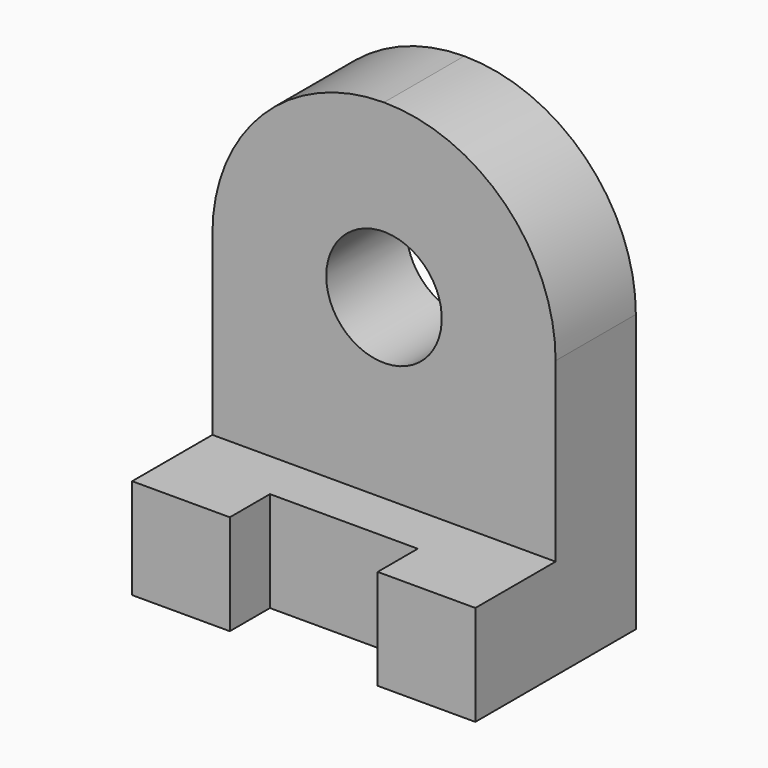
from build123d import *

# Parameters (mm, degrees)
F0_W     = 66.04
F0_H     = 86.36
F1_DEPTH = 19.304
F2_R     = 33.01999
F3_W     = 66.04
F3_H     = 19.304
F4_DEPTH = 19.304
F5_W     = 66.04
F5_H     = 19.304
F6_DEPTH = 9.652
F7_W     = 18.796
F7_H     = 19.304
F8_DEPTH = 9.652
F10_D    = 22.225


# Not quite as in the source:
# - a fillet or chamfer is up to 0.001 mm smaller than in the source, because OpenCascade refuses the exact size


with BuildPart() as f1:
    # F0 (on Front) → F1 (new body)
    with BuildSketch(Plane.XZ):
        with Locations((33.02, 43.18)):
            Rectangle(F0_W, F0_H)
    extrude(amount=F1_DEPTH)

    # F2 (radius 33.02 in the source; OpenCascade refuses exactly that, so slightly less here)
    f2_edges = [f1.edges().sort_by_distance(p)[0] for p in [
        (66.04, -9.652, 86.36),
        (0, -9.652, 86.36),
    ]]
    fillet(f2_edges, radius=F2_R)

    # F3 (on Front) → F4 (join)
    with BuildSketch(Plane.XZ):
        with Locations((33.02, 9.652)):
            Rectangle(F3_W, F3_H)
    extrude(amount=F4_DEPTH)

    # F5 (on face) → F6 (join)
    with BuildSketch(Plane.XZ.offset(19.304)):
        with Locations((33.02, 9.652)):
            Rectangle(F5_W, F5_H)
    extrude(amount=F6_DEPTH)

    # F7 (on face) → F8 (join)
    with BuildSketch(Plane.XZ.offset(28.956)):
        with Locations((9.398, 9.652)):
            Rectangle(F7_W, F7_H)
        with Locations((56.642, 9.652)):
            Rectangle(F7_W, F7_H)
    extrude(amount=F8_DEPTH)

    # F10 (through all)
    with Locations(Plane.XZ.offset(19.304)):
        with Locations((33.02, 53.34)):
            Hole(F10_D / 2)


solid = f1.part
